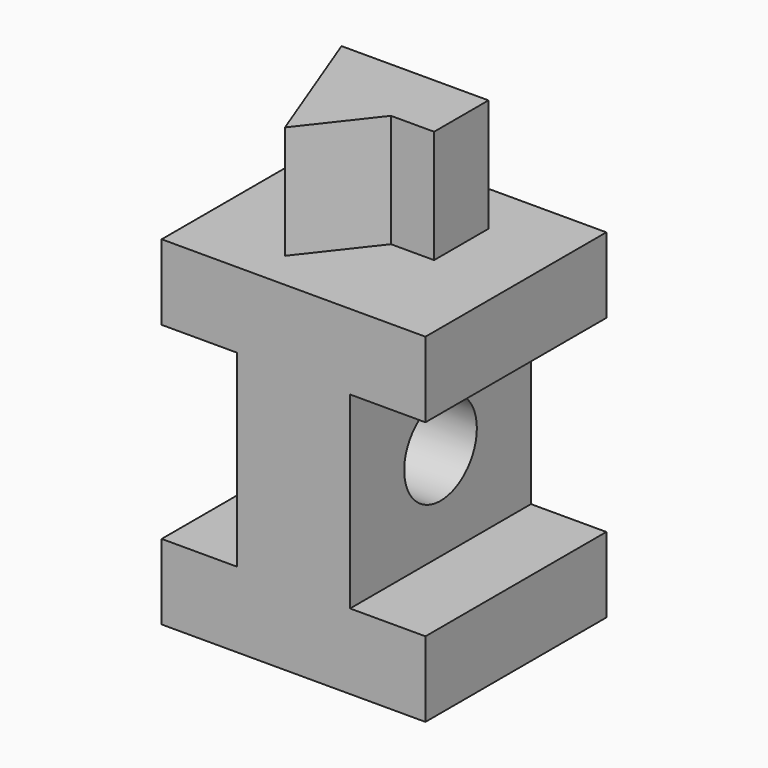
from build123d import *

# Parameters (mm, degrees)
F1_DEPTH = 76.2
F2_R     = 15.3048554067
F3_DEPTH = 63.501
F5_DEPTH = 38.1


# Not quite as in the source:
# - a feature names something its author has since deleted; it is built from what else it names


with BuildPart() as f1:
    # F0 (on Front) → F1 (new body)
    with BuildSketch(Plane.XZ):
        Polygon((-48.8696609855, -52.1779545115), (40.0303390145, -52.1779545115), (40.0303390145, -26.7779545115), (14.6303390145, -26.7779545115), (14.6303390145, 36.7220454885), (40.0303390145, 36.7220454885), (40.0303390145, 62.1220454885), (-48.8696609855, 62.1220454885), (-48.8696609855, 36.7220454885), (-23.4696609855, 36.7220454885), (-23.4696609855, -26.7779545115), (-48.8696609855, -26.7779545115), align=None)
    extrude(amount=F1_DEPTH)

    # F2 (on face) → F3 (cut, through all)
    with BuildSketch(Plane.YZ.offset(14.6303390145)):
        with Locations((-38.1, 4.9720454885)):
            Circle(F2_R)
    extrude(amount=-F3_DEPTH, mode=Mode.SUBTRACT)

    # F4 (on face) → F5 (join)
    with BuildSketch(Plane.XY.offset(62.1220454885)):
        Polygon((-17.6424384117, -63.2961168885), (0, -40.7014116645), (14.5472735167, -40.7014116645), (14.5472735167, -17.7971962839), (-34.9753573537, -17.7971962839), align=None)
    extrude(amount=F5_DEPTH)


solid = f1.part
